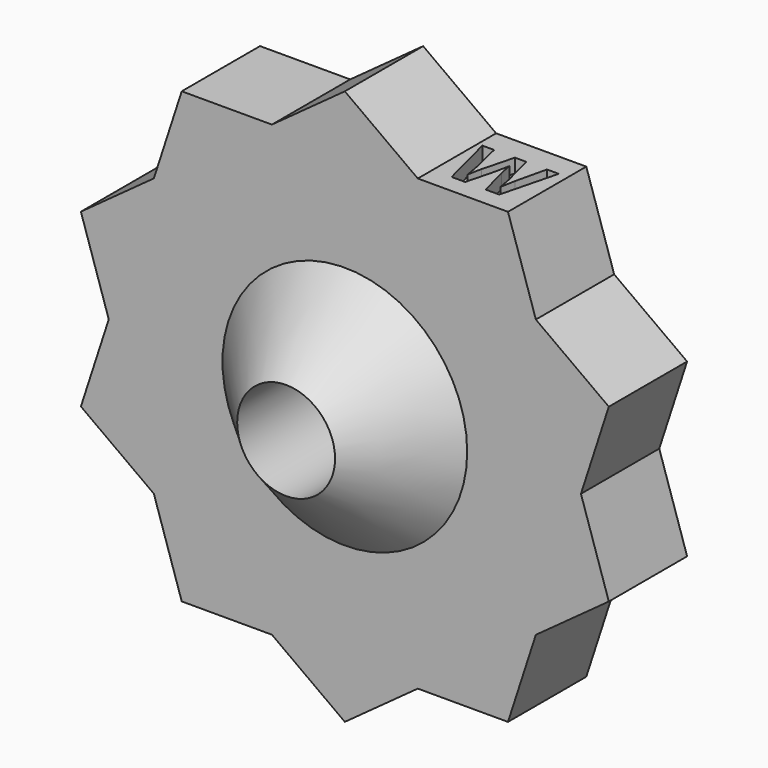
from build123d import *

# Parameters (mm, degrees)
F2_DEPTH      = 12
F3_DEPTH      = 12
F4_R          = 15
F5_DEPTH      = 9
F6_R          = 15
F7_DEPTH      = 9
F8_SIZE       = 8.99999
F9_SIZE       = 8.99999
F10_R         = 6.00001
F11_DEPTH     = 90
F12_TEXT_SIZE = 9.6925639861
F13_DEPTH     = 1.7


# Not quite as in the source:
# - a fillet or chamfer is up to 0.001 mm smaller than in the source, because OpenCascade refuses the exact size
# - Text() gives the source's letters only with a copy of the font that has no kerning and outlines rounded to 1/6400 em; it was checked with that copy


with BuildPart() as f2:
    # F0 (on Front) → F2 (new body)
    with BuildSketch(Plane.XZ):
        Polygon((20, 27.5276384094), (-20, 27.5276384094), (-32.360679775, -10.5146222424), (0, -34.0260323341), (32.360679775, -10.5146222424), align=None)
    extrude(amount=F2_DEPTH)

    # F1 (on Front) → F3 (join)
    with BuildSketch(Plane.XZ):
        Polygon((32.360679775, 10.5146222424), (0, 34.0260323341), (-32.360679775, 10.5146222424), (-20, -27.5276384094), (20, -27.5276384094), align=None)
    extrude(amount=F3_DEPTH)

    # F4 (on face) → F5 (join)
    with BuildSketch(Plane.XZ.offset(12)):
        Circle(F4_R)
    extrude(amount=F5_DEPTH)

    # F6 (on face) → F7 (join)
    with BuildSketch(Plane(origin=(0, 0, 0), x_dir=(-1, 0, 0), z_dir=(0, 1, 0))):
        Circle(F6_R)
    extrude(amount=F7_DEPTH)

    # F8 (size 9 in the source; OpenCascade refuses exactly that, so slightly less here)
    f8_edges = [f2.edges().sort_by_distance(p)[0] for p in [
        (15, 9, 0),
    ]]
    chamfer(f8_edges, length=F8_SIZE)

    # F9 (size 9 in the source; OpenCascade refuses exactly that, so slightly less here)
    f9_edges = [f2.edges().sort_by_distance(p)[0] for p in [
        (-15, -21, 0),
    ]]
    chamfer(f9_edges, length=F9_SIZE)

    # F10 (on face) → F11 (cut)
    with BuildSketch(Plane(origin=(0, 9, 0), x_dir=(-1, 0, 0), z_dir=(0, 1, 0))):
        Circle(F10_R)
    extrude(amount=-F11_DEPTH, mode=Mode.SUBTRACT)

    # F12 (on face) → F13 (cut)
    with BuildSketch(Plane.XY.offset(27.5276384094)):
        with Locations((9.5058245096, -9.7331723728)):
            Text('W', F12_TEXT_SIZE, font='Open Sans', font_style=FontStyle.BOLD, text_align=(TextAlign.LEFT, TextAlign.BOTTOM))
    extrude(amount=-F13_DEPTH, mode=Mode.SUBTRACT)


solid = f2.part
